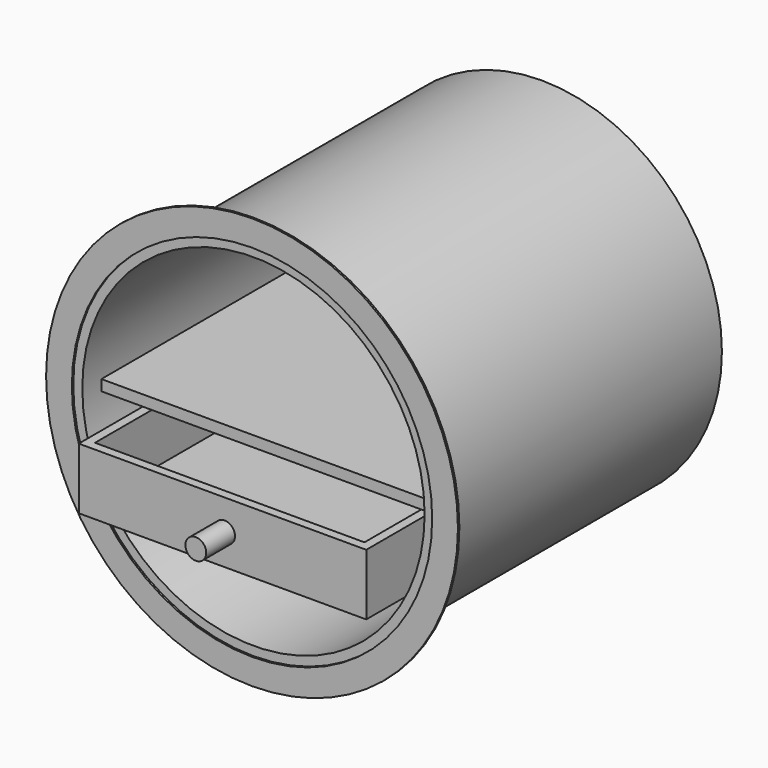
from build123d import *

# Parameters (mm, degrees)
F0_R         = 50
F1_DEPTH     = 100
F2_T         = -2.5
F3_W         = 94.1821336746
F3_H         = 77.1465990692
F4_DEPTH     = 3
F7_W         = 79.7765403986
F7_H         = 17.0111740008
F8_DEPTH     = 110
F9_R         = 2.8886289283
F10_DEPTH    = 10
F12_T        = 2.5
F12_T3_DEPTH = 22.0111740008
F12_T5_DEPTH = 84.7765403986
F13_R        = 57.146981612
F13_R_2      = 50
F14_DEPTH    = 0.5


# Not quite as in the source:
# - a shell that OpenCascade refuses in one call is made with other operations: the cavity is built on its own and cut out
# - a feature names something its author has since deleted; it is built from what else it names
# - the program builds the solid bodies; features that only make, move or delete a surface that nothing else refers to are left out


with BuildPart() as f1:
    # F0 (on Front) → F1 (new body)
    with BuildSketch(Plane.XZ):
        Circle(F0_R)
    extrude(amount=F1_DEPTH)

    # F2
    f2_openings = [f1.faces().sort_by_distance(p)[0] for p in [
        (0, -100, 0),
    ]]
    offset(amount=F2_T, openings=f2_openings)

    # F7 (on Front) → F8 (join)
    with BuildSketch(Plane.XZ):
        with Locations((-0.586591661, -15.6913413666)):
            Rectangle(F7_W, F7_H)
    extrude(amount=F8_DEPTH)

    # F9 (on face) → F10 (join)
    with BuildSketch(Plane.XZ.offset(110)):
        with Locations((0, -15.6913418323)):
            Circle(F9_R)
    extrude(amount=F10_DEPTH)

    # F12: shell of thickness 2.5, made by hand


with BuildPart() as f4:
    # F3 (on Top) → F4 (new body)
    with BuildSketch(Plane.XY):
        with Locations((0.1425482333, -55.4851768538)):
            Rectangle(F3_W, F3_H)
    extrude(amount=-F4_DEPTH)


with BuildPart() as f12_core1:
    # F12_t2: copy of F1
    add(f1.part)

    # the walls: a layer under each face that stays
    f12_faces = [f12_core1.faces().sort_by_distance(p)[0] for p in [
        (-50, -50, 0),
        (0, 0, 0),
        (-46.6666666667, -100, -13.3333333333),
        (-47.5, -51.25, 0),
        (0, -2.5, 0),
        (-40.4748618603, -56.25, -15.6913413666),
        (-0.586591661, -56.25, -24.196928367),
        (39.3016785383, -56.25, -15.6913413666),
        (-27.1787717938, -110, -21.3617327002),
        (-2.8886289283, -115, -15.6913418323),
        (0, -120, -15.6913418323),
    ]]
    thicken(f12_faces, amount=-F12_T, mode=Mode.SUBTRACT)

    # F12_s4 → F12_t3 (cut)
    with BuildSketch(Plane.XY.offset(-26.696928367)):
        Polygon((-40.4998618603, -2.525), (-40.4748618603, 0), (-37.9748618603, 0), (-37.9748618603, -2.5), align=None)
        Polygon((39.3266785383, -2.525), (39.3016785383, 0), (36.8016785383, 0), (36.8016785383, -2.5), align=None)
    extrude(amount=F12_T3_DEPTH, mode=Mode.SUBTRACT)

    # F12_s6 → F12_t5 (cut)
    with BuildSketch(Plane.YZ.offset(-42.9748618603)):
        Polygon((-2.525, -24.221928367), (0, -24.196928367), (0, -21.696928367), (-2.5, -21.696928367), align=None)
    extrude(amount=F12_T5_DEPTH, mode=Mode.SUBTRACT)

    # F12_s7 → F12_t8 (revolve, cut)
    with BuildSketch(Plane.XY):
        Polygon((47.475, -2.525), (50, -2.5), (50, 0), (47.5, 0), align=None)
    revolve(axis=Axis((0, -2.5, 0), (0, 1, 0)), mode=Mode.SUBTRACT)

    # F12_s9 → F12_t10 (revolve, cut)
    with BuildSketch(Plane.XY.offset(-15.6913418323)):
        Polygon((2.9136289283, -110.025), (2.8886289283, -107.5), (0.3886289283, -107.5), (0.3886289283, -110), align=None)
    revolve(axis=Axis((0, -110, -15.6913418323), (0, -1, 0)), mode=Mode.SUBTRACT)


with BuildPart() as f1_1:
    add(f1.part)

    # what is left inside the walls is the cavity
    f12_cavity = [f12_core1.part.solids().sort_by_distance(p)[0] for p in [
        (-0.586592, -72.5, -7.210754),
    ]]
    add(f12_cavity, mode=Mode.SUBTRACT)


with BuildPart() as f14:
    # F13 (on face) → F14 (new body)
    with BuildSketch(Plane.XZ.offset(100)):
        Circle(F13_R)
        Circle(F13_R_2, mode=Mode.SUBTRACT)
    extrude(amount=F14_DEPTH)


solid = Compound([f4.part, f1_1.part, f14.part])
